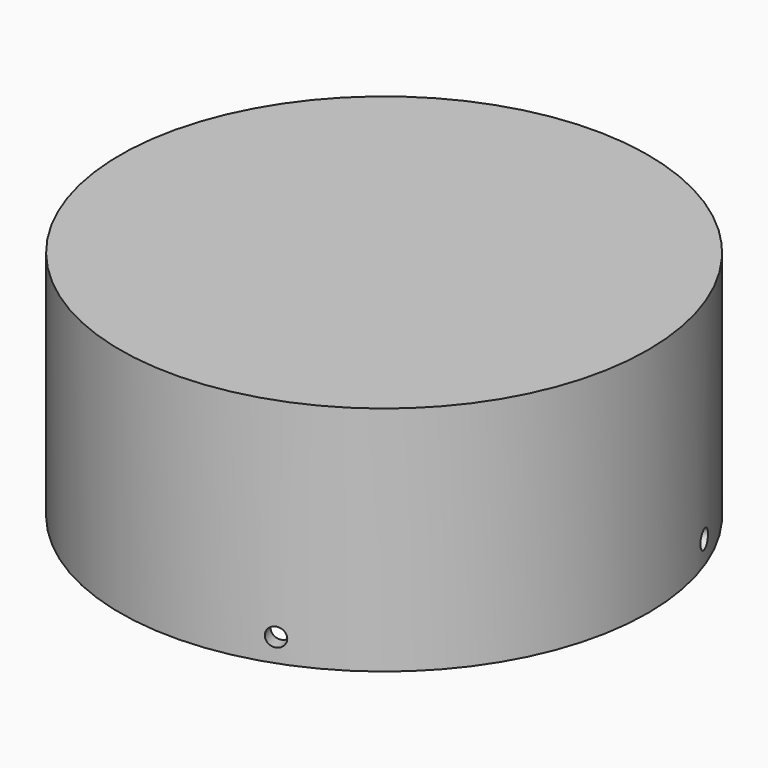
from build123d import *

# Parameters (mm, degrees)
F0_R            = 28.5
F1_DEPTH        = 25
F2_T            = -1.5
F6_D            = 2
F6_COPIES_COUNT = 2
F6_COPIES_ANGLE = 90


# Not quite as in the source:
# - a pattern or mirror of a feature is missing from the dataset's text; its kind, count and spacing are read off the source's solid


with BuildPart() as f1:
    # F0 (on Top) → F1 (new body)
    with BuildSketch(Plane.XY):
        Circle(F0_R)
    extrude(amount=F1_DEPTH)

    # F2
    f2_openings = [f1.faces().sort_by_distance(p)[0] for p in [
        (0, 0, 0),
    ]]
    offset(amount=F2_T, openings=f2_openings)

    # F6 (through all)
    with Locations(Plane(origin=(10.2606042998, -28.1907786236, 0), x_dir=(0.9396926208, 0.3420201433, 0), z_dir=(0.3420201433, -0.9396926208, 0))):
        with Locations((0, 2.5)):
            f6 = Hole(F6_D / 2)

    # F6_copies: F6 ×2 about axis
    f6_copies_axis = Axis((0, 0, 0), (0, 0, 1))
    for i in range(1, F6_COPIES_COUNT):
        add(f6.rotate(f6_copies_axis, i * F6_COPIES_ANGLE / (F6_COPIES_COUNT - 1)), mode=Mode.SUBTRACT)


solid = f1.part
